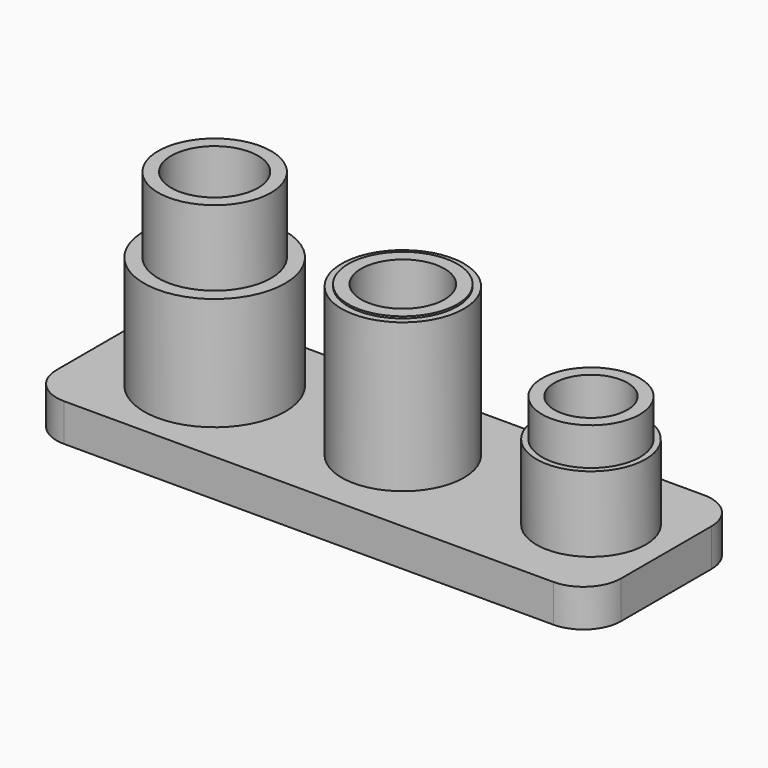
from build123d import *

# Parameters (mm, degrees)
F0_R     = 3
F0_R_2   = 2.9
F0_R_3   = 2.6
F1_DEPTH = 2
F0_R_4   = 2.31
F2_DEPTH = 12
F0_R_5   = 2.215
F3_DEPTH = 10
F0_R_6   = 1.94
F4_DEPTH = 8
F5_R     = 3.75
F5_R_2   = 3.25
F5_R_3   = 2.9
F6_DEPTH = 2
F5_R_4   = 2.215
F7_DEPTH = 6
F5_R_5   = 2.54
F8_DEPTH = 9.9
F5_R_6   = 2.835
F9_DEPTH = 8


with BuildPart() as f1:
    # F0 (on Top) → F1 (new body)
    with BuildSketch(Plane.XY):
        with BuildLine():
            Line((-12, -5), (12, -5))
            ThreePointArc((12, -5), (13.4142135624, -4.4142135624), (14, -3))
            Line((14, -3), (14, 3))
            ThreePointArc((14, 3), (13.4142135624, 4.4142135624), (12, 5))
            Line((12, 5), (-12, 5))
            ThreePointArc((-12, 5), (-13.4142135624, 4.4142135624), (-14, 3))
            Line((-14, 3), (-14, -3))
            ThreePointArc((-14, -3), (-13.4142135624, -4.4142135624), (-12, -5))
        make_face()
        with Locations((-10, 0)):
            Circle(F0_R, mode=Mode.SUBTRACT)
        Circle(F0_R_2, mode=Mode.SUBTRACT)
        with Locations((10, 0)):
            Circle(F0_R_3, mode=Mode.SUBTRACT)
    extrude(amount=F1_DEPTH)

    # F0 (on Top) → F2 (join)
    with BuildSketch(Plane.XY):
        with Locations((-10, 0)):
            Circle(F0_R)
        with Locations((-10, 0)):
            Circle(F0_R_4, mode=Mode.SUBTRACT)
    extrude(amount=F2_DEPTH)

    # F0 (on Top) → F3 (join)
    with BuildSketch(Plane.XY):
        Circle(F0_R_2)
        Circle(F0_R_5, mode=Mode.SUBTRACT)
    extrude(amount=F3_DEPTH)

    # F0 (on Top) → F4 (join)
    with BuildSketch(Plane.XY):
        with Locations((10, 0)):
            Circle(F0_R_3)
        with Locations((10, 0)):
            Circle(F0_R_6, mode=Mode.SUBTRACT)
    extrude(amount=F4_DEPTH)


with BuildPart() as f6:
    # F5 (on Top) → F6 (new body)
    with BuildSketch(Plane.XY):
        with BuildLine():
            Line((-12, -5), (12, -5))
            ThreePointArc((12, -5), (13.4142135624, -4.4142135624), (14, -3))
            Line((14, -3), (14, 3))
            ThreePointArc((14, 3), (13.4142135624, 4.4142135624), (12, 5))
            Line((12, 5), (-12, 5))
            Line((-12, 5), (-14, 5))
            ThreePointArc((-14, 5), (-15.4142135624, 4.4142135624), (-16, 3))
            Line((-16, 3), (-16, -3))
            ThreePointArc((-16, -3), (-15.4142135624, -4.4142135624), (-14, -5))
            Line((-14, -5), (-12, -5))
        make_face()
        with Locations((-10, 0)):
            Circle(F5_R, mode=Mode.SUBTRACT)
        Circle(F5_R_2, mode=Mode.SUBTRACT)
        with Locations((10, 0)):
            Circle(F5_R_3, mode=Mode.SUBTRACT)
    extrude(amount=F6_DEPTH)

    # F5 (on Top) → F7 (join)
    with BuildSketch(Plane.XY):
        with Locations((10, 0)):
            Circle(F5_R_3)
        with Locations((10, 0)):
            Circle(F5_R_4, mode=Mode.SUBTRACT)
    extrude(amount=F7_DEPTH)

    # F5 (on Top) → F8 (join)
    with BuildSketch(Plane.XY):
        Circle(F5_R_2)
        Circle(F5_R_5, mode=Mode.SUBTRACT)
    extrude(amount=F8_DEPTH)

    # F5 (on Top) → F9 (join)
    with BuildSketch(Plane.XY):
        with Locations((-10, 0)):
            Circle(F5_R)
        with Locations((-10, 0)):
            Circle(F5_R_6, mode=Mode.SUBTRACT)
    extrude(amount=F9_DEPTH)


solid = Compound([f1.part, f6.part])
